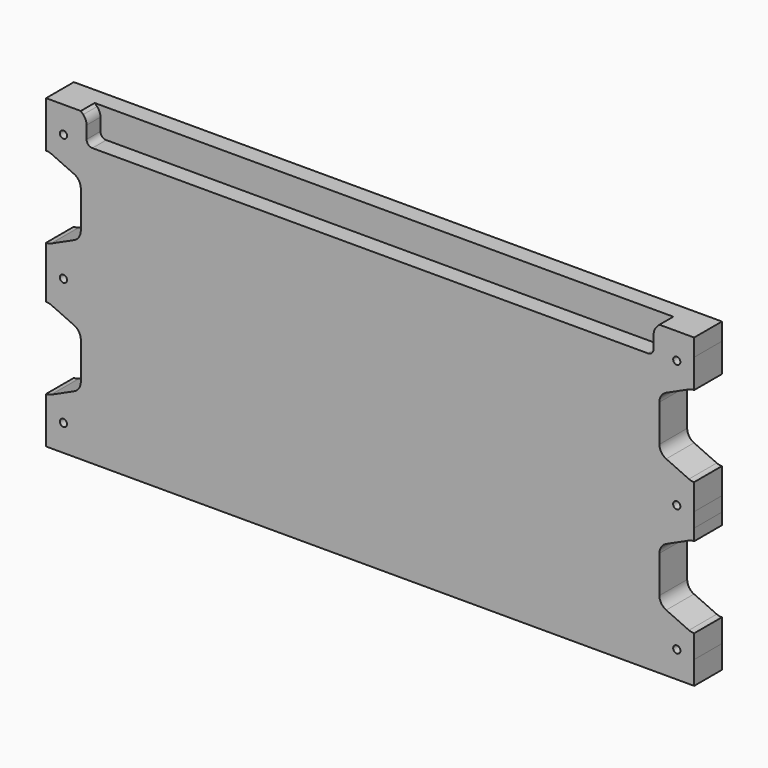
from build123d import *

# Parameters (mm, degrees)
F0_R      = 1.984375
F1_DEPTH  = 9.525
F1_FACE_R = 1.984375
F2_DEPTH  = 9.525
F3_SIZE   = 3.175
F4_R      = 6.35


# Not quite as in the source:
# - ends of sketch curves that miss each other by under 0.0002 mm in the source are joined
# - a feature names something its author has since deleted; it is built from what else it names


with BuildPart() as f1:
    # F0 (on Front) → F1 (new body)
    with BuildSketch(Plane.XZ):
        with BuildLine():
            Line((141.6844258, 36.003738), (149.2250254, 36.003738))
            Line((149.2250254, 36.003738), (149.2250254, 47.116238))
            Line((149.2250254, 47.116238), (149.2250254, 50.291238))
            Line((149.2250254, 50.291238), (149.0129496538, 50.291238))
            ThreePointArc((149.0129496538, 50.291238), (147.6686550901, 50.4351625794), (146.3852981737, 50.8604121335))
            Line((146.3852981737, 50.8604121335), (133.8973485199, 56.5367601413))
            ThreePointArc((133.8973485199, 56.5367601413), (131.1860821837, 58.8797877952), (130.175, 62.3175860078))
            Line((130.175, 62.3175860078), (130.175, 82.7148899922))
            ThreePointArc((130.175, 82.7148899922), (131.1860821837, 86.1526882048), (133.8973485199, 88.4957158587))
            Line((133.8973485199, 88.4957158587), (146.3852981737, 94.1720638665))
            ThreePointArc((146.3852981737, 94.1720638665), (147.6686550901, 94.5973134206), (149.0129496538, 94.741238))
            Line((149.0129496538, 94.741238), (149.225, 94.741238))
            Line((149.225, 94.741238), (149.2250254, 110.616238))
            Line((149.2250254, 110.616238), (149.2250254, 120.141238))
            Line((149.2250254, 120.141238), (127.0000254, 120.141238))
            Line((127.0000254, 120.141238), (127.0000254, 107.441238))
            ThreePointArc((127.0000254, 107.441238), (126.0700894303, 105.1961739697), (123.8250254, 104.266238))
            Line((123.8250254, 104.266238), (-180.9749746, 104.266238))
            ThreePointArc((-180.9749746, 104.266238), (-183.2200386303, 105.1961739697), (-184.1499746, 107.441238))
            Line((-184.1499746, 107.441238), (-184.1499746, 120.141238))
            Line((-184.1499746, 120.141238), (-206.3749746, 120.141238))
            Line((-206.3749746, 120.141238), (-206.3749746, 94.741238))
            Line((-206.3749746, 94.741238), (-206.1629496538, 94.741238))
            ThreePointArc((-206.1629496538, 94.741238), (-204.8186550901, 94.5973134206), (-203.5352981737, 94.1720638665))
            Line((-203.5352981737, 94.1720638665), (-191.0473485199, 88.4957158587))
            ThreePointArc((-191.0473485199, 88.4957158587), (-188.3360821837, 86.1526882048), (-187.325, 82.7148899922))
            Line((-187.325, 82.7148899922), (-187.325, 62.3175860078))
            ThreePointArc((-187.325, 62.3175860078), (-188.3360821837, 58.8797877952), (-191.0473485199, 56.5367601413))
            Line((-191.0473485199, 56.5367601413), (-203.5352981737, 50.8604121335))
            ThreePointArc((-203.5352981737, 50.8604121335), (-204.8186550901, 50.4351625794), (-206.1629496538, 50.291238))
            Line((-206.1629496538, 50.291238), (-206.375, 50.291238))
            Line((-206.375, 50.291238), (-206.3749746, 36.003738))
            Line((-206.3749746, 36.003738), (-198.834375, 36.003738))
            ThreePointArc((-198.834375, 36.003738), (-196.85, 37.988113), (-194.865625, 36.003738))
            Line((-194.865625, 36.003738), (137.7156758, 36.003738))
            ThreePointArc((137.7156758, 36.003738), (139.7000508, 37.988113), (141.6844258, 36.003738))
        make_face()
        with Locations((-196.8500060797, 105.6372644242)):
            Circle(F0_R, mode=Mode.SUBTRACT)
        with Locations((139.7000060797, 105.853738)):
            Circle(F0_R, mode=Mode.SUBTRACT)
        with BuildLine():
            Line((149.225, 21.716238), (149.225, 28.066238))
            Line((149.225, 28.066238), (149.2250254, 36.003738))
            Line((149.2250254, 36.003738), (141.6844258, 36.003738))
            ThreePointArc((141.6844258, 36.003738), (139.7000508, 34.019363), (137.7156758, 36.003738))
            Line((137.7156758, 36.003738), (-194.865625, 36.003738))
            ThreePointArc((-194.865625, 36.003738), (-196.85, 34.019363), (-198.834375, 36.003738))
            Line((-198.834375, 36.003738), (-206.3749746, 36.003738))
            Line((-206.3749746, 36.003738), (-206.3749746, 21.716238))
            Line((-206.3749746, 21.716238), (-206.1629496538, 21.716238))
            ThreePointArc((-206.1629496538, 21.716238), (-204.8186550901, 21.5723134206), (-203.5352981737, 21.1470638665))
            Line((-203.5352981737, 21.1470638665), (-191.0473485199, 15.4707158587))
            ThreePointArc((-191.0473485199, 15.4707158587), (-188.3360821837, 13.1276882048), (-187.325, 9.6898899922))
            Line((-187.325, 9.6898899922), (-187.325, -10.7074139922))
            ThreePointArc((-187.325, -10.7074139922), (-188.3360821837, -14.1452122048), (-191.0473485199, -16.4882398587))
            Line((-191.0473485199, -16.4882398587), (-203.5352981737, -22.1645878665))
            ThreePointArc((-203.5352981737, -22.1645878665), (-204.8186550901, -22.5898374206), (-206.1629496538, -22.733762))
            Line((-206.1629496538, -22.733762), (-206.375, -22.733762))
            Line((-206.375, -22.733762), (-206.3749746, -48.133762))
            Line((-206.3749746, -48.133762), (149.2250254, -48.133762))
            Line((149.2250254, -48.133762), (149.2250254, -35.433762))
            Line((149.2250254, -35.433762), (149.225, -22.733762))
            Line((149.225, -22.733762), (149.0129496538, -22.733762))
            ThreePointArc((149.0129496538, -22.733762), (147.6686550901, -22.5898374206), (146.3852981737, -22.1645878665))
            Line((146.3852981737, -22.1645878665), (133.8973485199, -16.4882398587))
            ThreePointArc((133.8973485199, -16.4882398587), (131.1860821837, -14.1452122048), (130.175, -10.7074139922))
            Line((130.175, -10.7074139922), (130.175, 9.6898899922))
            ThreePointArc((130.175, 9.6898899922), (131.1860821837, 13.1276882048), (133.8973485199, 15.4707158587))
            Line((133.8973485199, 15.4707158587), (146.3852981737, 21.1470638665))
            ThreePointArc((146.3852981737, 21.1470638665), (147.6686550901, 21.5723134206), (149.0129496538, 21.716238))
            Line((149.0129496538, 21.716238), (149.225, 21.716238))
        make_face()
        with Locations((-196.8500060797, -33.6297884242)):
            Circle(F0_R, mode=Mode.SUBTRACT)
        with Locations((139.7000060797, -33.6297884242)):
            Circle(F0_R, mode=Mode.SUBTRACT)
    extrude(amount=F1_DEPTH)

    # F0 (on Front) + F1_face (on face) → F2 (join)
    with BuildSketch(Plane.XZ):
        with BuildLine():
            Line((149.225, 21.716238), (149.225, 28.066238))
            Line((149.225, 28.066238), (149.2250254, 36.003738))
            Line((149.2250254, 36.003738), (141.6844258, 36.003738))
            ThreePointArc((141.6844258, 36.003738), (139.7000508, 34.019363), (137.7156758, 36.003738))
            Line((137.7156758, 36.003738), (-194.865625, 36.003738))
            ThreePointArc((-194.865625, 36.003738), (-196.85, 34.019363), (-198.834375, 36.003738))
            Line((-198.834375, 36.003738), (-206.3749746, 36.003738))
            Line((-206.3749746, 36.003738), (-206.3749746, 21.716238))
            Line((-206.3749746, 21.716238), (-206.1629496538, 21.716238))
            ThreePointArc((-206.1629496538, 21.716238), (-204.8186550901, 21.5723134206), (-203.5352981737, 21.1470638665))
            Line((-203.5352981737, 21.1470638665), (-191.0473485199, 15.4707158587))
            ThreePointArc((-191.0473485199, 15.4707158587), (-188.3360821837, 13.1276882048), (-187.325, 9.6898899922))
            Line((-187.325, 9.6898899922), (-187.325, -10.7074139922))
            ThreePointArc((-187.325, -10.7074139922), (-188.3360821837, -14.1452122048), (-191.0473485199, -16.4882398587))
            Line((-191.0473485199, -16.4882398587), (-203.5352981737, -22.1645878665))
            ThreePointArc((-203.5352981737, -22.1645878665), (-204.8186550901, -22.5898374206), (-206.1629496538, -22.733762))
            Line((-206.1629496538, -22.733762), (-206.375, -22.733762))
            Line((-206.375, -22.733762), (-206.3749746, -48.133762))
            Line((-206.3749746, -48.133762), (149.2250254, -48.133762))
            Line((149.2250254, -48.133762), (149.2250254, -35.433762))
            Line((149.2250254, -35.433762), (149.225, -22.733762))
            Line((149.225, -22.733762), (149.0129496538, -22.733762))
            ThreePointArc((149.0129496538, -22.733762), (147.6686550901, -22.5898374206), (146.3852981737, -22.1645878665))
            Line((146.3852981737, -22.1645878665), (133.8973485199, -16.4882398587))
            ThreePointArc((133.8973485199, -16.4882398587), (131.1860821837, -14.1452122048), (130.175, -10.7074139922))
            Line((130.175, -10.7074139922), (130.175, 9.6898899922))
            ThreePointArc((130.175, 9.6898899922), (131.1860821837, 13.1276882048), (133.8973485199, 15.4707158587))
            Line((133.8973485199, 15.4707158587), (146.3852981737, 21.1470638665))
            ThreePointArc((146.3852981737, 21.1470638665), (147.6686550901, 21.5723134206), (149.0129496538, 21.716238))
            Line((149.0129496538, 21.716238), (149.225, 21.716238))
        make_face()
        with Locations((-196.8500060797, -33.6297884242)):
            Circle(F0_R, mode=Mode.SUBTRACT)
        with Locations((139.7000060797, -33.6297884242)):
            Circle(F0_R, mode=Mode.SUBTRACT)
        with BuildLine():
            Line((141.6844258, 36.003738), (149.2250254, 36.003738))
            Line((149.2250254, 36.003738), (149.2250254, 47.116238))
            Line((149.2250254, 47.116238), (149.2250254, 50.291238))
            Line((149.2250254, 50.291238), (149.0129496538, 50.291238))
            ThreePointArc((149.0129496538, 50.291238), (147.6686550901, 50.4351625794), (146.3852981737, 50.8604121335))
            Line((146.3852981737, 50.8604121335), (133.8973485199, 56.5367601413))
            ThreePointArc((133.8973485199, 56.5367601413), (131.1860821837, 58.8797877952), (130.175, 62.3175860078))
            Line((130.175, 62.3175860078), (130.175, 82.7148899922))
            ThreePointArc((130.175, 82.7148899922), (131.1860821837, 86.1526882048), (133.8973485199, 88.4957158587))
            Line((133.8973485199, 88.4957158587), (146.3852981737, 94.1720638665))
            ThreePointArc((146.3852981737, 94.1720638665), (147.6686550901, 94.5973134206), (149.0129496538, 94.741238))
            Line((149.0129496538, 94.741238), (149.225, 94.741238))
            Line((149.225, 94.741238), (149.2250254, 110.616238))
            Line((149.2250254, 110.616238), (149.2250254, 120.141238))
            Line((149.2250254, 120.141238), (127.0000254, 120.141238))
            Line((127.0000254, 120.141238), (127.0000254, 107.441238))
            ThreePointArc((127.0000254, 107.441238), (126.0700894303, 105.1961739697), (123.8250254, 104.266238))
            Line((123.8250254, 104.266238), (-180.9749746, 104.266238))
            ThreePointArc((-180.9749746, 104.266238), (-183.2200386303, 105.1961739697), (-184.1499746, 107.441238))
            Line((-184.1499746, 107.441238), (-184.1499746, 120.141238))
            Line((-184.1499746, 120.141238), (-206.3749746, 120.141238))
            Line((-206.3749746, 120.141238), (-206.3749746, 94.741238))
            Line((-206.3749746, 94.741238), (-206.1629496538, 94.741238))
            ThreePointArc((-206.1629496538, 94.741238), (-204.8186550901, 94.5973134206), (-203.5352981737, 94.1720638665))
            Line((-203.5352981737, 94.1720638665), (-191.0473485199, 88.4957158587))
            ThreePointArc((-191.0473485199, 88.4957158587), (-188.3360821837, 86.1526882048), (-187.325, 82.7148899922))
            Line((-187.325, 82.7148899922), (-187.325, 62.3175860078))
            ThreePointArc((-187.325, 62.3175860078), (-188.3360821837, 58.8797877952), (-191.0473485199, 56.5367601413))
            Line((-191.0473485199, 56.5367601413), (-203.5352981737, 50.8604121335))
            ThreePointArc((-203.5352981737, 50.8604121335), (-204.8186550901, 50.4351625794), (-206.1629496538, 50.291238))
            Line((-206.1629496538, 50.291238), (-206.375, 50.291238))
            Line((-206.375, 50.291238), (-206.3749746, 36.003738))
            Line((-206.3749746, 36.003738), (-198.834375, 36.003738))
            ThreePointArc((-198.834375, 36.003738), (-196.85, 37.988113), (-194.865625, 36.003738))
            Line((-194.865625, 36.003738), (137.7156758, 36.003738))
            ThreePointArc((137.7156758, 36.003738), (139.7000508, 37.988113), (141.6844258, 36.003738))
        make_face()
        with Locations((-196.8500060797, 105.6372644242)):
            Circle(F0_R, mode=Mode.SUBTRACT)
        with Locations((139.7000060797, 105.853738)):
            Circle(F0_R, mode=Mode.SUBTRACT)
        with BuildLine():
            Line((127.0000254, 107.441238), (127.0000254, 120.141238))
            Line((127.0000254, 120.141238), (-184.1499746, 120.141238))
            Line((-184.1499746, 120.141238), (-184.1499746, 107.441238))
            ThreePointArc((-184.1499746, 107.441238), (-183.2200386303, 105.1961739697), (-180.9749746, 104.266238))
            Line((-180.9749746, 104.266238), (123.8250254, 104.266238))
            ThreePointArc((123.8250254, 104.266238), (126.0700894303, 105.1961739697), (127.0000254, 107.441238))
        make_face()
    with BuildSketch(Plane(origin=(-28.5749924989, -9.525, 28.7740351311), x_dir=(1, 0, 0), z_dir=(0, -1, 0))):
        with BuildLine():
            Line((177.7999924989, -0.7077971311), (177.8000178989, 7.2297028689))
            Line((177.8000178989, 7.2297028689), (177.8000178989, 21.5172028689))
            Line((177.8000178989, 21.5172028689), (177.5879421527, 21.5172028689))
            ThreePointArc((177.5879421527, 21.5172028689), (176.2436475891, 21.6611274483), (174.9602906726, 22.0863770023))
            Line((174.9602906726, 22.0863770023), (162.4723410188, 27.7627250102))
            ThreePointArc((162.4723410188, 27.7627250102), (159.7610746826, 30.1057526641), (158.7499924989, 33.5435508767))
            Line((158.7499924989, 33.5435508767), (158.7499924989, 53.940854861))
            ThreePointArc((158.7499924989, 53.940854861), (159.7610746826, 57.3786530736), (162.4723410188, 59.7216807275))
            Line((162.4723410188, 59.7216807275), (174.9602906726, 65.3980287354))
            ThreePointArc((174.9602906726, 65.3980287354), (176.2436475891, 65.8232782895), (177.5879421527, 65.9672028689))
            Line((177.5879421527, 65.9672028689), (177.7999924989, 65.9672028689))
            Line((177.7999924989, 65.9672028689), (177.8000178989, 81.8422028689))
            Line((177.8000178989, 81.8422028689), (177.8000178989, 91.3672028689))
            Line((177.8000178989, 91.3672028689), (155.5750178989, 91.3672028689))
            Line((155.5750178989, 91.3672028689), (155.5750178989, 78.6672028689))
            ThreePointArc((155.5750178989, 78.6672028689), (154.6450819292, 76.4221388386), (152.4000178989, 75.4922028689))
            Line((152.4000178989, 75.4922028689), (-152.3999821011, 75.4922028689))
            ThreePointArc((-152.3999821011, 75.4922028689), (-154.6450461313, 76.4221388386), (-155.5749821011, 78.6672028689))
            Line((-155.5749821011, 78.6672028689), (-155.5749821011, 91.3672028689))
            Line((-155.5749821011, 91.3672028689), (-177.7999821011, 91.3672028689))
            Line((-177.7999821011, 91.3672028689), (-177.7999821011, 65.9672028689))
            Line((-177.7999821011, 65.9672028689), (-177.5879571548, 65.9672028689))
            ThreePointArc((-177.5879571548, 65.9672028689), (-176.2436625912, 65.8232782895), (-174.9603056747, 65.3980287354))
            Line((-174.9603056747, 65.3980287354), (-162.472356021, 59.7216807275))
            ThreePointArc((-162.472356021, 59.7216807275), (-159.7610896847, 57.3786530736), (-158.7500075011, 53.940854861))
            Line((-158.7500075011, 53.940854861), (-158.7500075011, 33.5435508767))
            ThreePointArc((-158.7500075011, 33.5435508767), (-159.7610896847, 30.1057526641), (-162.472356021, 27.7627250102))
            Line((-162.472356021, 27.7627250102), (-174.9603056747, 22.0863770023))
            ThreePointArc((-174.9603056747, 22.0863770023), (-176.2436625912, 21.6611274483), (-177.5879571548, 21.5172028689))
            Line((-177.5879571548, 21.5172028689), (-177.8000075011, 21.5172028689))
            Line((-177.8000075011, 21.5172028689), (-177.7999821011, 7.2297028689))
            Line((-177.7999821011, 7.2297028689), (-177.7999821011, -7.0577971311))
            Line((-177.7999821011, -7.0577971311), (-177.5879571548, -7.0577971311))
            ThreePointArc((-177.5879571548, -7.0577971311), (-176.2436625912, -7.2017217105), (-174.9603056747, -7.6269712646))
            Line((-174.9603056747, -7.6269712646), (-162.472356021, -13.3033192725))
            ThreePointArc((-162.472356021, -13.3033192725), (-159.7610896847, -15.6463469264), (-158.7500075011, -19.084145139))
            Line((-158.7500075011, -19.084145139), (-158.7500075011, -39.4814491233))
            ThreePointArc((-158.7500075011, -39.4814491233), (-159.7610896847, -42.9192473359), (-162.472356021, -45.2622749898))
            Line((-162.472356021, -45.2622749898), (-174.9603056747, -50.9386229977))
            ThreePointArc((-174.9603056747, -50.9386229977), (-176.2436625912, -51.3638725517), (-177.5879571548, -51.5077971311))
            Line((-177.5879571548, -51.5077971311), (-177.8000075011, -51.5077971311))
            Line((-177.8000075011, -51.5077971311), (-177.7999821011, -76.9077971311))
            Line((-177.7999821011, -76.9077971311), (177.8000178989, -76.9077971311))
            Line((177.8000178989, -76.9077971311), (177.8000178989, -64.2077971311))
            Line((177.8000178989, -64.2077971311), (177.7999924989, -51.5077971311))
            Line((177.7999924989, -51.5077971311), (177.5879421527, -51.5077971311))
            ThreePointArc((177.5879421527, -51.5077971311), (176.2436475891, -51.3638725517), (174.9602906726, -50.9386229977))
            Line((174.9602906726, -50.9386229977), (162.4723410188, -45.2622749898))
            ThreePointArc((162.4723410188, -45.2622749898), (159.7610746826, -42.9192473359), (158.7499924989, -39.4814491233))
            Line((158.7499924989, -39.4814491233), (158.7499924989, -19.084145139))
            ThreePointArc((158.7499924989, -19.084145139), (159.7610746826, -15.6463469264), (162.4723410188, -13.3033192725))
            Line((162.4723410188, -13.3033192725), (174.9602906726, -7.6269712646))
            ThreePointArc((174.9602906726, -7.6269712646), (176.2436475891, -7.2017217105), (177.5879421527, -7.0577971311))
            Line((177.5879421527, -7.0577971311), (177.7999924989, -7.0577971311))
            Line((177.7999924989, -7.0577971311), (177.7999924989, -0.7077971311))
        make_face()
        with Locations((168.2750432989, 7.2297028689)):
            Circle(F1_FACE_R, mode=Mode.SUBTRACT)
        with Locations((-168.2750075011, 7.2297028689)):
            Circle(F1_FACE_R, mode=Mode.SUBTRACT)
        with Locations((-168.2750135807, -62.4038235553)):
            Circle(F1_FACE_R, mode=Mode.SUBTRACT)
        with Locations((168.2749985786, -62.4038235553)):
            Circle(F1_FACE_R, mode=Mode.SUBTRACT)
        with Locations((168.2749985786, 77.0797028689)):
            Circle(F1_FACE_R, mode=Mode.SUBTRACT)
        with Locations((-168.2750135807, 76.8632292931)):
            Circle(F1_FACE_R, mode=Mode.SUBTRACT)
    extrude(amount=-F2_DEPTH)

    # F3
    f3_edges = [f1.edges().sort_by_distance(p)[0] for p in [
        (-184.149975, -4.7625, 120.141238),
        (127.000025, -4.7625, 120.141238),
    ]]
    chamfer(f3_edges, length=F3_SIZE)

    # F4
    f4_edges = [f1.edges().sort_by_distance(p)[0] for p in [
        (-184.149975, -4.7625, 116.966238),
        (127.000025, -4.7625, 116.966238),
    ]]
    fillet(f4_edges, radius=F4_R)


solid = f1.part
